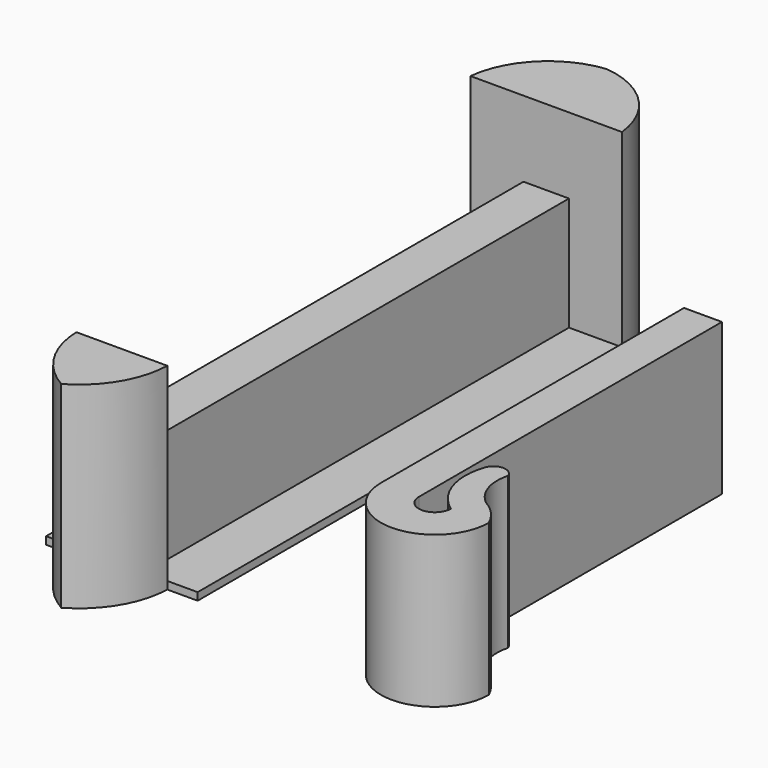
from build123d import *

# Parameters (mm, degrees)
F0_W     = 3
F0_H     = 29.6977118962
F0_H_2   = 40.3022881038
F1_DEPTH = 1
F2_DEPTH = 15
F3_DEPTH = 25
F4_W     = 5
F4_H     = 50
F5_DEPTH = 20


# Not quite as in the source:
# - ends of sketch curves that miss each other by under 0.0002 mm in the source are joined


with BuildPart() as f1:
    # F0 (on Top) → F1 (new body)
    with BuildSketch(Plane.XY):
        with BuildLine():
            Line((-3, 35), (0, 35))
            Line((0, 35), (0, 45))
            ThreePointArc((0, 45), (-6.7636906533, 41.7636906533), (-10, 35))
            Line((-10, 35), (-3, 35))
        make_face()
        with BuildLine():
            Line((0, 45), (0, 35))
            Line((0, 35), (3, 35))
            Line((3, 35), (10, 35))
            ThreePointArc((10, 35), (6.7636906533, 41.7636906533), (0, 45))
        make_face()
        with Locations((-1.5, 20.1511440519)):
            Rectangle(F0_W, F0_H)
        with Locations((-1.5, -14.8488559481)):
            Rectangle(F0_W, F0_H_2)
        with BuildLine():
            Line((3, -35), (0, -35))
            Line((0, -35), (0, -45))
            ThreePointArc((0, -45), (4.3065233729, -40.7839140238), (6, -35))
            Line((6, -35), (3, -35))
        make_face()
        Polygon((10, 35), (3, 35), (3, -35), (6, -35), (10, -35), align=None)
        Polygon((3, 35), (0, 35), (0, 5.3022881038), (0, -35), (3, -35), align=None)
        Polygon((-3, 5.3022881038), (-3, 35), (-10, 35), (-10, -35), (-6, -35), (-3, -35), align=None)
        with BuildLine():
            Line((0, -45), (0, -35))
            Line((0, -35), (-3, -35))
            Line((-3, -35), (-6, -35))
            ThreePointArc((-6, -35), (-4.3065233729, -40.7839140238), (0, -45))
        make_face()
    extrude(amount=-F1_DEPTH)

    # F0 (on Top) → F2 (join)
    with BuildSketch(Plane.XY):
        with Locations((-1.5, -14.8488559481)):
            Rectangle(F0_W, F0_H_2)
        Polygon((3, 35), (0, 35), (0, 5.3022881038), (0, -35), (3, -35), align=None)
        with Locations((-1.5, 20.1511440519)):
            Rectangle(F0_W, F0_H)
    extrude(amount=F2_DEPTH)

    # F0 (on Top) → F3 (join)
    with BuildSketch(Plane.XY):
        with BuildLine():
            Line((-3, 35), (0, 35))
            Line((0, 35), (0, 45))
            ThreePointArc((0, 45), (-6.7636906533, 41.7636906533), (-10, 35))
            Line((-10, 35), (-3, 35))
        make_face()
        with BuildLine():
            Line((0, 45), (0, 35))
            Line((0, 35), (3, 35))
            Line((3, 35), (10, 35))
            ThreePointArc((10, 35), (6.7636906533, 41.7636906533), (0, 45))
        make_face()
        with BuildLine():
            Line((0, -45), (0, -35))
            Line((0, -35), (-3, -35))
            Line((-3, -35), (-6, -35))
            ThreePointArc((-6, -35), (-4.3065233729, -40.7839140238), (0, -45))
        make_face()
        with BuildLine():
            Line((3, -35), (0, -35))
            Line((0, -35), (0, -45))
            ThreePointArc((0, -45), (4.3065233729, -40.7839140238), (6, -35))
            Line((6, -35), (3, -35))
        make_face()
    extrude(amount=F3_DEPTH)


with BuildPart() as f5:
    # F4 (on Top) → F5 (new body)
    with BuildSketch(Plane.XY):
        with BuildLine():
            Line((38.5142476857, -34.1587369061), (33.5142476857, -34.1587369061))
            ThreePointArc((33.5142476857, -34.1587369061), (40.6328371912, -41.2773264116), (47.7514266968, -34.1587369061))
            ThreePointArc((47.7514266968, -34.1587369061), (46.4966279337, -32.249134599), (44.7070300579, -30.8284163475))
            ThreePointArc((44.7070300579, -30.8284163475), (42.8230618595, -28.0632723139), (42.7514279717, -24.7180927545))
            ThreePointArc((42.7514279717, -24.7180927545), (41.2503035036, -23.6761727856), (39.7491790354, -24.7180927545))
            ThreePointArc((39.7491790354, -24.7180927545), (39.6705937247, -29.9407833051), (42.7514279717, -34.1587369061))
            ThreePointArc((42.7514279717, -34.1587369061), (40.6328371912, -36.2773276865), (38.5142476857, -34.1587369061))
        make_face()
        with Locations((36.0142476857, -9.1587369061)):
            Rectangle(F4_W, F4_H)
    extrude(amount=F5_DEPTH)


solid = Compound([f1.part, f5.part])
